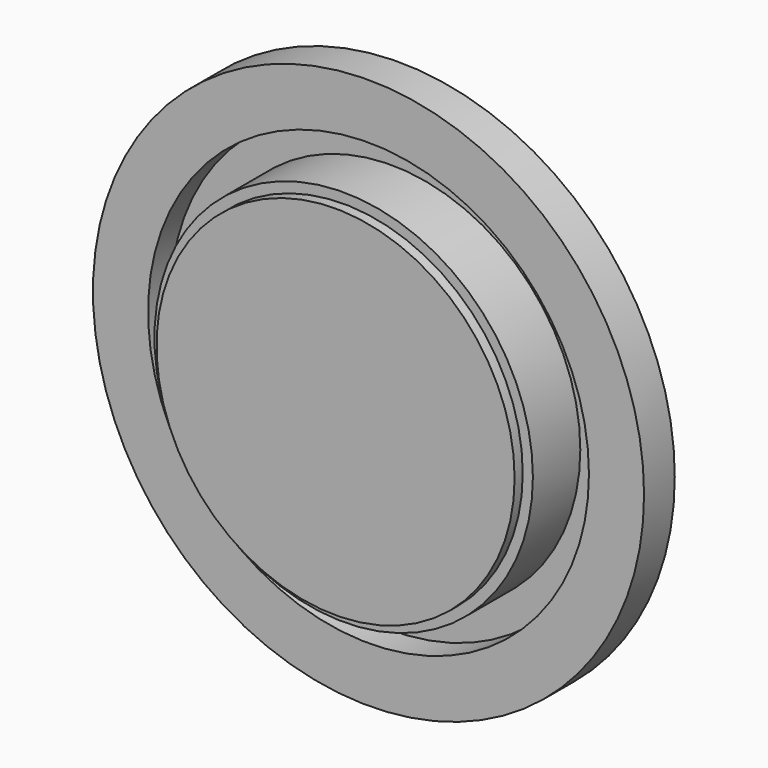
from build123d import *

# Parameters (mm, degrees)
F0_W     = 1.57
F0_H     = 0.51
F3_R     = 9
F4_DEPTH = 0.51


# Not quite as in the source:
# - the program builds the solid bodies; features that only make, move or delete a surface that nothing else refers to are left out


with BuildPart() as f1:
    # F0 (on Top) → F1 (revolve)
    with BuildSketch(Plane.XY):
        Polygon((9, 3.49), (9, 0), (9.51, 0), (9.51, 2.98), (9.51, 3.49), align=None)
        with Locations((10.295, 3.235)):
            Rectangle(F0_W, F0_H)
        Polygon((13.85, 3.49), (11.08, 3.49), (11.08, 2.98), (11.08, 1.56), (13.85, 1.56), align=None)
    revolve(axis=Axis((0, 1.745, 0), (0, 1, 0)))

    # F3 (on offset) → F4 (join)
    with BuildSketch(Plane.XZ):
        Circle(F3_R)
    extrude(amount=F4_DEPTH)


solid = f1.part
